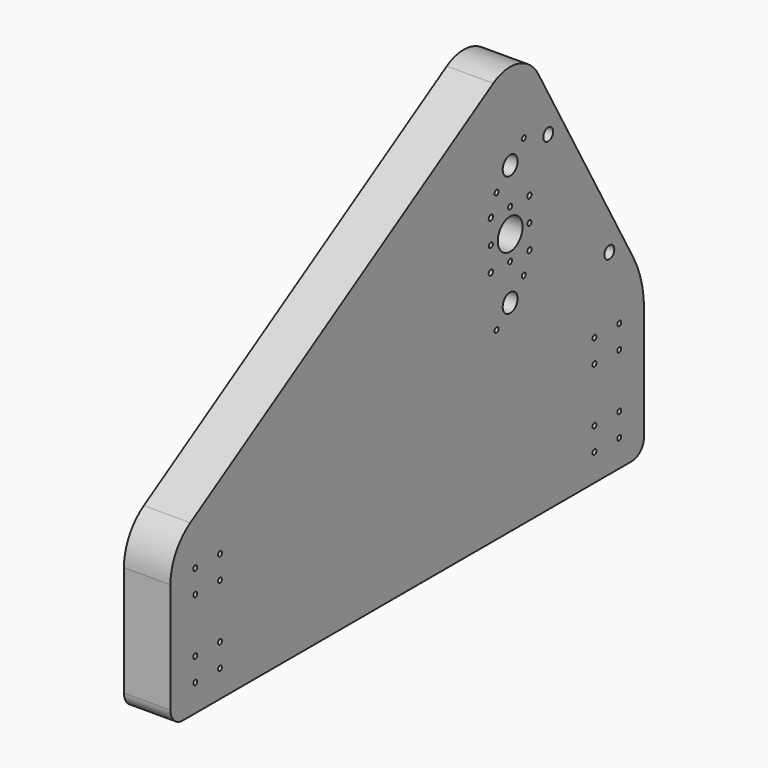
from build123d import *

# Parameters (mm, degrees)
F0_R     = 1.6
F0_R_2   = 6
F0_R_3   = 4
F0_R_4   = 1.75
F0_R_5   = 10
F1_DEPTH = 30


# Not quite as in the source:
# - ends of sketch curves that miss each other by under 0.0002 mm in the source are joined


with BuildPart() as f1:
    # F0 (on Right) → F1 (new body)
    with BuildSketch(Plane.YZ):
        with BuildLine():
            Line((191, -122.083788), (191, -49.632945))
            ThreePointArc((191, -49.632945), (188.7918883648, -32.5816457168), (182.3132286148, -16.6552672181))
            Line((182.3132286148, -16.6552672181), (112.877133, 106))
            Line((112.877133, 106), (105.625999, 118.808753))
            ThreePointArc((105.625999, 118.808753), (89.4861101441, 131.177974009), (69.378816691, 128.1464075024))
            Line((69.378816691, 128.1464075024), (-174.970501, -22.141031))
            ThreePointArc((-174.970501, -22.141031), (-186.7206628889, -34.3919513631), (-191, -50.818717))
            Line((-191, -50.818717), (-191, -122.083788))
            ThreePointArc((-191, -122.083788), (-188.0956097489, -129.0956087489), (-181.083789, -132))
            Line((-181.083789, -132), (83, -132))
            Line((83, -132), (181.083788, -132))
            ThreePointArc((181.083788, -132), (188.0956087489, -129.0956087489), (191, -122.083788))
        make_face()
        with Locations((-171, -114.5)):
            Circle(F0_R, mode=Mode.SUBTRACT)
        with Locations((-171, -99.5)):
            Circle(F0_R, mode=Mode.SUBTRACT)
        with Locations((-151, -114.5)):
            Circle(F0_R, mode=Mode.SUBTRACT)
        with Locations((-151, -99.5)):
            Circle(F0_R, mode=Mode.SUBTRACT)
        with Locations((-171, -64.5)):
            Circle(F0_R, mode=Mode.SUBTRACT)
        with Locations((-151, -64.5)):
            Circle(F0_R, mode=Mode.SUBTRACT)
        with Locations((-171, -49.5)):
            Circle(F0_R, mode=Mode.SUBTRACT)
        with Locations((-151, -49.5)):
            Circle(F0_R, mode=Mode.SUBTRACT)
        with Locations((151, -114.5)):
            Circle(F0_R, mode=Mode.SUBTRACT)
        with Locations((151, -99.5)):
            Circle(F0_R, mode=Mode.SUBTRACT)
        with Locations((171, -114.5)):
            Circle(F0_R, mode=Mode.SUBTRACT)
        with Locations((171, -99.5)):
            Circle(F0_R, mode=Mode.SUBTRACT)
        with Locations((72.000954, -12.999046)):
            Circle(F0_R, mode=Mode.SUBTRACT)
        with Locations((83, -2)):
            Circle(F0_R_2, mode=Mode.SUBTRACT)
        with Locations((151, -64.5)):
            Circle(F0_R, mode=Mode.SUBTRACT)
        with Locations((171, -64.5)):
            Circle(F0_R, mode=Mode.SUBTRACT)
        with Locations((151, -49.5)):
            Circle(F0_R, mode=Mode.SUBTRACT)
        with Locations((171, -49.5)):
            Circle(F0_R, mode=Mode.SUBTRACT)
        with Locations((162.986451, -5.858929)):
            Circle(F0_R_3, mode=Mode.SUBTRACT)
        with Locations((93.999046, 8.999046)):
            Circle(F0_R, mode=Mode.SUBTRACT)
        with Locations((67.443651, 21.443651)):
            Circle(F0_R_4, mode=Mode.SUBTRACT)
        with Locations((83, 21.445)):
            Circle(F0_R, mode=Mode.SUBTRACT)
        with Locations((67.445, 37)):
            Circle(F0_R, mode=Mode.SUBTRACT)
        with Locations((83, 37)):
            Circle(F0_R_5, mode=Mode.SUBTRACT)
        with Locations((67.443651, 52.556349)):
            Circle(F0_R_4, mode=Mode.SUBTRACT)
        with Locations((83, 52.555)):
            Circle(F0_R, mode=Mode.SUBTRACT)
        with Locations((72.000954, 65.000954)):
            Circle(F0_R, mode=Mode.SUBTRACT)
        with Locations((98.556349, 21.443651)):
            Circle(F0_R_4, mode=Mode.SUBTRACT)
        with Locations((98.555, 37)):
            Circle(F0_R, mode=Mode.SUBTRACT)
        with Locations((98.556349, 52.556349)):
            Circle(F0_R_4, mode=Mode.SUBTRACT)
        with Locations((83, 76)):
            Circle(F0_R_2, mode=Mode.SUBTRACT)
        with Locations((93.999046, 86.999046)):
            Circle(F0_R, mode=Mode.SUBTRACT)
        with Locations((113.720248, 81.167269)):
            Circle(F0_R_3, mode=Mode.SUBTRACT)
    extrude(amount=F1_DEPTH)


solid = f1.part
